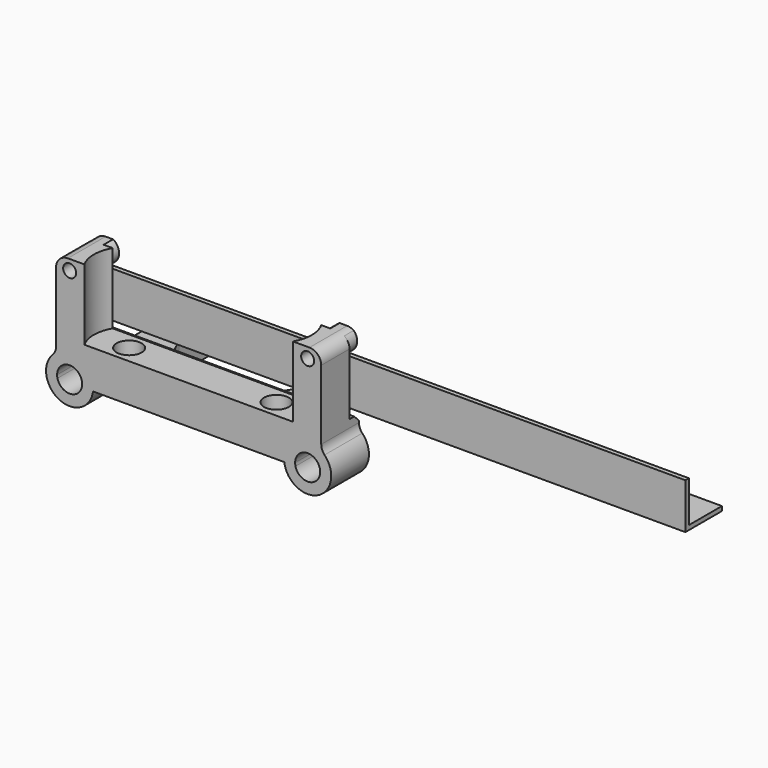
from build123d import *
from build123d import SkipClean  # not in build123d's __all__

# Parameters (mm, degrees)
F1_DEPTH      = 200
F2_R          = 4.25
F3_DEPTH      = 12
F3_DEPTH_BACK = 1
F4_DEPTH      = 25
F5_R          = 2.2
F6_DEPTH      = 25
F7_DEPTH      = 4
F8_DEPTH      = 12
F9_DEPTH      = 25
F10_DEPTH     = 4
F12_DEPTH     = 25
F14_DEPTH     = 8.7699061669
F13_R         = 2.2
F15_DEPTH     = 25
F16_T1_DEPTH  = 8.7699061669
F16_T6_DEPTH  = 15.8923048454
F16_S7_R      = 12
F16_T8_DEPTH  = 10
F16_T12_DEPTH = 15.8923048454
F16_S13_R     = 12
F16_T14_DEPTH = 10
F16_T19_DEPTH = 23.3923048454
F16_T23_DEPTH = 21.2699061669
F16_T31_DEPTH = 21.2699061669
F16_T36_DEPTH = 23.3923048454
F17_SIZE      = 2
F18_R         = 4


# Not quite as in the source:
# - a fillet or chamfer that OpenCascade refuses, or shapes differently, is made with other operations: its cross-section is extruded or revolved along the edge and cut away or added


with BuildPart() as f1:
    # F0 (on Right) → F1 (new body)
    with BuildSketch(Plane.YZ):
        Polygon((0, 15.5), (0, 0), (15.5, 0), (15.5, 1.5), (1.5, 1.5), (1.5, 15.5), align=None)
    extrude(amount=F1_DEPTH)


with BuildPart() as f3:
    # F2 (on Top) → F3 (new body, two sides)
    with BuildSketch(Plane.XY) as f3_sk:
        with BuildLine():
            Line((9.6076951546, -5), (0, -5))
            Line((0, -5), (0, -17))
            Line((0, -17), (9.6076951546, -17))
            ThreePointArc((9.6076951546, -17), (8, -11), (9.6076951546, -5))
        make_face()
        with BuildLine():
            Line((59.6076951546, -5), (30.3923048454, -5))
            ThreePointArc((30.3923048454, -5), (31.5911099155, -7.8941714588), (32, -11))
            ThreePointArc((32, -11), (31.5911099155, -14.1058285412), (30.3923048454, -17))
            Line((30.3923048454, -17), (59.6076951546, -17))
            ThreePointArc((59.6076951546, -17), (58, -11), (59.6076951546, -5))
        make_face()
        with BuildLine():
            Line((90, -5), (80.3923048454, -5))
            ThreePointArc((80.3923048454, -5), (81.5911099155, -7.8941714588), (82, -11))
            ThreePointArc((82, -11), (81.5911099155, -14.1058285412), (80.3923048454, -17))
            Line((80.3923048454, -17), (90, -17))
            Line((90, -17), (90, -5))
        make_face()
        with BuildLine():
            Line((30.3923048454, -5), (9.6076951546, -5))
            ThreePointArc((9.6076951546, -5), (8, -11), (9.6076951546, -17))
            Line((9.6076951546, -17), (30.3923048454, -17))
            ThreePointArc((30.3923048454, -17), (31.5911099155, -14.1058285412), (32, -11))
            ThreePointArc((32, -11), (31.5911099155, -7.8941714588), (30.3923048454, -5))
        make_face()
        with Locations((20, -11)):
            Circle(F2_R, mode=Mode.SUBTRACT)
        with BuildLine():
            Line((80.3923048454, -5), (59.6076951546, -5))
            ThreePointArc((59.6076951546, -5), (58, -11), (59.6076951546, -17))
            Line((59.6076951546, -17), (80.3923048454, -17))
            ThreePointArc((80.3923048454, -17), (81.5911099155, -14.1058285412), (82, -11))
            ThreePointArc((82, -11), (81.5911099155, -7.8941714588), (80.3923048454, -5))
        make_face()
        with Locations((70, -11)):
            Circle(F2_R, mode=Mode.SUBTRACT)
    extrude(amount=-F3_DEPTH)
    extrude(f3_sk.sketch, amount=F3_DEPTH_BACK)

    # F2 (on Top) → F4 (join)
    with BuildSketch(Plane.XY):
        with BuildLine():
            Line((9.6076951546, -5), (0, -5))
            Line((0, -5), (0, -17))
            Line((0, -17), (9.6076951546, -17))
            ThreePointArc((9.6076951546, -17), (8, -11), (9.6076951546, -5))
        make_face()
        with BuildLine():
            Line((90, -5), (80.3923048454, -5))
            ThreePointArc((80.3923048454, -5), (81.5911099155, -7.8941714588), (82, -11))
            ThreePointArc((82, -11), (81.5911099155, -14.1058285412), (80.3923048454, -17))
            Line((80.3923048454, -17), (90, -17))
            Line((90, -17), (90, -5))
        make_face()
    extrude(amount=F4_DEPTH)

    # F5 (on face) → F6 (cut)
    with BuildSketch(Plane(origin=(0, -5, 0), x_dir=(-1, 0, 0), z_dir=(0, 1, 0))):
        with Locations((-4.6076951546, 21.5)):
            Circle(F5_R)
        with Locations((-85.3923048454, 21.5)):
            Circle(F5_R)
    extrude(amount=-F6_DEPTH, mode=Mode.SUBTRACT)

    # F5 (on face) → F7 (join)
    with BuildSketch(Plane(origin=(0, -5, 0), x_dir=(-1, 0, 0), z_dir=(0, 1, 0))):
        with BuildLine():
            ThreePointArc((-0.6076951546, 21.5), (-1.1619755859, 23.5315060063), (-2.6712034815, 25))
            Line((-2.6712034815, 25), (-6.5441868277, 25))
            ThreePointArc((-6.5441868277, 25), (-6.6392011609, 18.0542804313), (-0.6076951546, 21.5))
        make_face()
        with Locations((-4.6076951546, 21.5)):
            Circle(F5_R, mode=Mode.SUBTRACT)
        with BuildLine():
            ThreePointArc((-81.3923048454, 21.5), (-81.9465852767, 23.5315060063), (-83.4558131723, 25))
            Line((-83.4558131723, 25), (-87.3287965185, 25))
            ThreePointArc((-87.3287965185, 25), (-87.4238108518, 18.0542804313), (-81.3923048454, 21.5))
        make_face()
        with Locations((-85.3923048454, 21.5)):
            Circle(F5_R, mode=Mode.SUBTRACT)
    extrude(amount=F7_DEPTH)

    # F5 (on face) → F8 (join, through all)
    with BuildSketch(Plane(origin=(0, -5, 0), x_dir=(-1, 0, 0), z_dir=(0, 1, 0))):
        with BuildLine():
            ThreePointArc((3.3923048454, -11), (2.4937681185, -7.3163578646), (0, -4.4601876661))
            Line((0, -4.4601876661), (0, -12))
            Line((0, -12), (-0.4770172441, -12))
            ThreePointArc((-0.4770172441, -12), (-4.6076951546, -15.25), (-8.7383730651, -12))
            Line((-8.7383730651, -12), (-12.5449490878, -12))
            ThreePointArc((-12.5449490878, -12), (-4.1067118542, -18.9842980739), (3.3923048454, -11))
        make_face()
        with BuildLine():
            Line((-90, -12), (-90, -4.4601876661))
            ThreePointArc((-90, -4.4601876661), (-89.5134312597, -17.8568445423), (-77.4550509122, -12))
            Line((-77.4550509122, -12), (-81.2616269349, -12))
            ThreePointArc((-81.2616269349, -12), (-85.3923048454, -15.25), (-89.5229827559, -12))
            Line((-89.5229827559, -12), (-90, -12))
        make_face()
        with BuildLine():
            ThreePointArc((-77.3923048454, -11), (-81.70866271, -3.898536727), (-90, -4.4601876661))
            Line((-90, -4.4601876661), (-90, -12))
            Line((-90, -12), (-89.5229827559, -12))
            ThreePointArc((-89.5229827559, -12), (-85.8958517055, -6.7799359531), (-81.1423048454, -11))
            ThreePointArc((-81.1423048454, -11), (-81.1722407985, -11.50354686), (-81.2616269349, -12))
            Line((-81.2616269349, -12), (-77.4550509122, -12))
            ThreePointArc((-77.4550509122, -12), (-77.4080067715, -11.5009833003), (-77.3923048454, -11))
        make_face()
    extrude(amount=-F8_DEPTH)

    # F5 (on face) → F9 (cut)
    with BuildSketch(Plane(origin=(0, -5, 0), x_dir=(-1, 0, 0), z_dir=(0, 1, 0))):
        with BuildLine():
            Line((-89.5229827559, -12), (-81.2616269349, -12))
            ThreePointArc((-81.2616269349, -12), (-81.1722407985, -11.50354686), (-81.1423048454, -11))
            ThreePointArc((-81.1423048454, -11), (-85.8958517055, -6.7799359531), (-89.5229827559, -12))
        make_face()
        with BuildLine():
            ThreePointArc((-0.3576951546, -11), (-5.1112420146, -6.7799359531), (-8.7383730651, -12))
            Line((-8.7383730651, -12), (-0.4770172441, -12))
            ThreePointArc((-0.4770172441, -12), (-0.3876311077, -11.50354686), (-0.3576951546, -11))
        make_face()
    with SkipClean():  # cleaning this boolean's faces spoils the solid; the shape is the same uncleaned
        extrude(amount=-F9_DEPTH, mode=Mode.SUBTRACT)

    # F5 (on face) → F10 (join)
    with BuildSketch(Plane(origin=(0, -5, 0), x_dir=(-1, 0, 0), z_dir=(0, 1, 0))):
        with BuildLine():
            Line((0, -4.4601876661), (0, 0))
            Line((0, 0), (-90, 0))
            Line((-90, 0), (-90, -4.4601876661))
            ThreePointArc((-90, -4.4601876661), (-81.70866271, -3.898536727), (-77.3923048454, -11))
            ThreePointArc((-77.3923048454, -11), (-77.4080067715, -11.5009833003), (-77.4550509122, -12))
            Line((-77.4550509122, -12), (-12.5449490878, -12))
            ThreePointArc((-12.5449490878, -12), (-8.7288215689, -4.1431554577), (0, -4.4601876661))
        make_face()
        with BuildLine():
            ThreePointArc((-77.3923048454, -11), (-81.70866271, -3.898536727), (-90, -4.4601876661))
            Line((-90, -4.4601876661), (-90, -12))
            Line((-90, -12), (-89.5229827559, -12))
            ThreePointArc((-89.5229827559, -12), (-85.8958517055, -6.7799359531), (-81.1423048454, -11))
            ThreePointArc((-81.1423048454, -11), (-81.1722407985, -11.50354686), (-81.2616269349, -12))
            Line((-81.2616269349, -12), (-77.4550509122, -12))
            ThreePointArc((-77.4550509122, -12), (-77.4080067715, -11.5009833003), (-77.3923048454, -11))
        make_face()
        with BuildLine():
            Line((-90, -12), (-90, -4.4601876661))
            ThreePointArc((-90, -4.4601876661), (-89.5134312597, -17.8568445423), (-77.4550509122, -12))
            Line((-77.4550509122, -12), (-81.2616269349, -12))
            ThreePointArc((-81.2616269349, -12), (-85.3923048454, -15.25), (-89.5229827559, -12))
            Line((-89.5229827559, -12), (-90, -12))
        make_face()
        with BuildLine():
            Line((0, -12), (0, -4.4601876661))
            ThreePointArc((0, -4.4601876661), (-8.7288215689, -4.1431554577), (-12.5449490878, -12))
            Line((-12.5449490878, -12), (-8.7383730651, -12))
            ThreePointArc((-8.7383730651, -12), (-5.1112420146, -6.7799359531), (-0.3576951546, -11))
            ThreePointArc((-0.3576951546, -11), (-0.3876311077, -11.50354686), (-0.4770172441, -12))
            Line((-0.4770172441, -12), (0, -12))
        make_face()
        with BuildLine():
            ThreePointArc((3.3923048454, -11), (2.4937681185, -7.3163578646), (0, -4.4601876661))
            Line((0, -4.4601876661), (0, -12))
            Line((0, -12), (-0.4770172441, -12))
            ThreePointArc((-0.4770172441, -12), (-4.6076951546, -15.25), (-8.7383730651, -12))
            Line((-8.7383730651, -12), (-12.5449490878, -12))
            ThreePointArc((-12.5449490878, -12), (-4.1067118542, -18.9842980739), (3.3923048454, -11))
        make_face()
    with SkipClean():  # cleaning this boolean's faces spoils the solid; the shape is the same uncleaned
        extrude(amount=F10_DEPTH)

    # F11 (on face) → F12 (join)
    with BuildSketch(Plane(origin=(0, -1, 0), x_dir=(-1, 0, 0), z_dir=(0, 1, 0))):
        with BuildLine():
            ThreePointArc((-77.2015328535, -2.2300938331), (-74.3857326292, -6.2192711802), (-73.3923048454, -11))
            Line((-73.3923048454, -11), (-65, -11))
            Line((-65, -11), (-65, -2.2300938331))
            Line((-65, -2.2300938331), (-77.2015328535, -2.2300938331))
        make_face()
        with BuildLine():
            Line((-25, -2.2300938331), (-25, -11))
            Line((-25, -11), (-16.6076951546, -11))
            ThreePointArc((-16.6076951546, -11), (-15.6142673708, -6.2192711802), (-12.7984671465, -2.2300938331))
            Line((-12.7984671465, -2.2300938331), (-25, -2.2300938331))
        make_face()
    extrude(amount=F12_DEPTH)

    # F13 (on face) → F14 (join, through all)
    with BuildSketch(Plane.XY.offset(-2.2300938331)):
        with BuildLine():
            Line((65, 15.5), (73.3923048454, 15.5))
            Line((73.3923048454, 15.5), (73.3923048454, 24))
            Line((73.3923048454, 24), (71.9912373946, 24))
            ThreePointArc((71.9912373946, 24), (72.6992987688, 22.8380828366), (72.9461524227, 21.5))
            ThreePointArc((72.9461524227, 21.5), (67.8580695861, 17.9968536539), (66.4010674508, 24))
            Line((66.4010674508, 24), (65, 24))
            Line((65, 24), (65, 15.5))
        make_face()
        with BuildLine():
            Line((66.4010674508, 24), (71.9912373946, 24))
            ThreePointArc((71.9912373946, 24), (69.1961524227, 25.25), (66.4010674508, 24))
        make_face()
        with BuildLine():
            Line((18.0087626054, 24), (23.5989325492, 24))
            ThreePointArc((23.5989325492, 24), (20.8038475773, 25.25), (18.0087626054, 24))
        make_face()
    extrude(amount=-F14_DEPTH)

    # F13 (on face) → F15 (cut)
    with BuildSketch(Plane.XY.offset(-2.2300938331)):
        with Locations((20.8038475773, 21.5)):
            Circle(F13_R)
        with Locations((69.1961524227, 21.5)):
            Circle(F13_R)
    extrude(amount=-F15_DEPTH, mode=Mode.SUBTRACT)

    # F16: fillet of radius 5 on 4 edges, made by hand

    # F16_s2 → F16_t1 (join)
    with BuildSketch(Plane.XY.offset(-11)):
        with BuildLine():
            ThreePointArc((60, -1), (63.5355339059, 0.4644660941), (65, 4))
            Line((65, 4), (65, -1))
            Line((65, -1), (60, -1))
        make_face()
        with BuildLine():
            ThreePointArc((30, -1), (26.4644660941, 0.4644660941), (25, 4))
            Line((25, 4), (25, -1))
            Line((25, -1), (30, -1))
        make_face()
    extrude(amount=F16_T1_DEPTH)


with BuildPart() as f16_tool4:
    # F16_s5 → F16_t6 (new body)
    with BuildSketch(Plane.YZ.offset(80.8923048454)):
        with BuildLine():
            ThreePointArc((-1, -12), (0.4188611699, -11.2565835097), (2, -11))
            Line((2, -11), (-1, -11))
            Line((-1, -11), (-1, -12))
        make_face()
    extrude(amount=-F16_T6_DEPTH)

    # F16_s7 → F16_t8 (cut, symmetric)
    with BuildSketch(Plane.XZ.offset(-0.5)):
        with Locations((85.3923048454, -11)):
            Circle(F16_S7_R)
    extrude(amount=F16_T8_DEPTH, both=True, mode=Mode.SUBTRACT)


with BuildPart() as f3_1:
    add(f3.part, clean=False)

    # F16_t3: union F16_tool4
    add(f16_tool4.part)


with BuildPart() as f16_tool10:
    # F16_s11 → F16_t12 (new body)
    with BuildSketch(Plane.YZ.offset(25)):
        with BuildLine():
            ThreePointArc((-1, -12), (0.4188611699, -11.2565835097), (2, -11))
            Line((2, -11), (-1, -11))
            Line((-1, -11), (-1, -12))
        make_face()
    extrude(amount=-F16_T12_DEPTH)

    # F16_s13 → F16_t14 (cut, symmetric)
    with BuildSketch(Plane.XZ.offset(-0.5)):
        with Locations((4.6076951546, -11)):
            Circle(F16_S13_R)
    extrude(amount=F16_T14_DEPTH, both=True, mode=Mode.SUBTRACT)


with BuildPart() as f3_2:
    add(f3_1.part, clean=False)

    # F16_t9: union F16_tool10
    add(f16_tool10.part)


with BuildPart() as f16_tool17:
    # F16_s18 → F16_t19 (new body)
    with BuildSketch(Plane.YZ.offset(80.8923048454)):
        with BuildLine():
            ThreePointArc((-1, -12), (0.4188611699, -11.2565835097), (2, -11))
            Line((2, -11), (-1, -11))
            Line((-1, -11), (-1, -12))
        make_face()
    extrude(amount=-F16_T19_DEPTH)

    split(bisect_by=Plane.YZ.offset(65), keep=Keep.BOTTOM)


with BuildPart() as f16_tool21:
    # F16_s22 → F16_t23 (new body)
    with BuildSketch(Plane.XY.offset(-23.5)):
        with BuildLine():
            ThreePointArc((60, -1), (63.5355339059, 0.4644660941), (65, 4))
            Line((65, 4), (65, -1))
            Line((65, -1), (60, -1))
        make_face()
    extrude(amount=F16_T23_DEPTH)

    split(bisect_by=Plane.XY.offset(-12), keep=Keep.TOP)

    split(bisect_by=Plane.XY.offset(-11), keep=Keep.BOTTOM)


with BuildPart() as f16_tool17_1:
    add(f16_tool17.part, clean=False)

    # F16_t26: intersect F16_tool21
    add(f16_tool21.part, mode=Mode.INTERSECT)


with BuildPart() as f3_3:
    add(f3_2.part, clean=False)

    # F16_t15: union F16_tool17
    add(f16_tool17_1.part)


with BuildPart() as f16_tool29:
    # F16_s30 → F16_t31 (new body)
    with BuildSketch(Plane.XY.offset(-2.2300938331)):
        with BuildLine():
            ThreePointArc((30, -1), (26.4644660941, 0.4644660941), (25, 4))
            Line((25, 4), (25, -1))
            Line((25, -1), (30, -1))
        make_face()
    extrude(amount=-F16_T31_DEPTH)

    split(bisect_by=Plane.XY.offset(-12), keep=Keep.TOP)

    split(bisect_by=Plane.XY.offset(-11), keep=Keep.BOTTOM)


with BuildPart() as f16_tool34:
    # F16_s35 → F16_t36 (new body)
    with BuildSketch(Plane.YZ.offset(32.5)):
        with BuildLine():
            ThreePointArc((-1, -12), (0.4188611699, -11.2565835097), (2, -11))
            Line((2, -11), (-1, -11))
            Line((-1, -11), (-1, -12))
        make_face()
    extrude(amount=-F16_T36_DEPTH)

    split(bisect_by=Plane.YZ.offset(25), keep=Keep.TOP)


with BuildPart() as f16_tool29_1:
    add(f16_tool29.part, clean=False)

    # F16_t38: intersect F16_tool34
    add(f16_tool34.part, mode=Mode.INTERSECT)


with BuildPart() as f3_4:
    add(f3_3.part, clean=False)

    # F16_t27: union F16_tool29
    add(f16_tool29_1.part)

    # F17
    f17_edges = [f3_4.edges().sort_by_distance(p)[0] for p in [
        (45, -1, 0),
    ]]
    chamfer(f17_edges, length=F17_SIZE)

    # F18
    f18_edges = [f3_4.edges().sort_by_distance(p)[0] for p in [
        (0, -11, -4.460188),
        (0, -3, -4.460188),
        (90, -3, -4.460188),
        (90, -11, 25),
        (0, -11, 25),
        (90, -11, -4.460188),
    ]]
    fillet(f18_edges, radius=F18_R)


solid = Compound([f1.part, f3_4.part])
